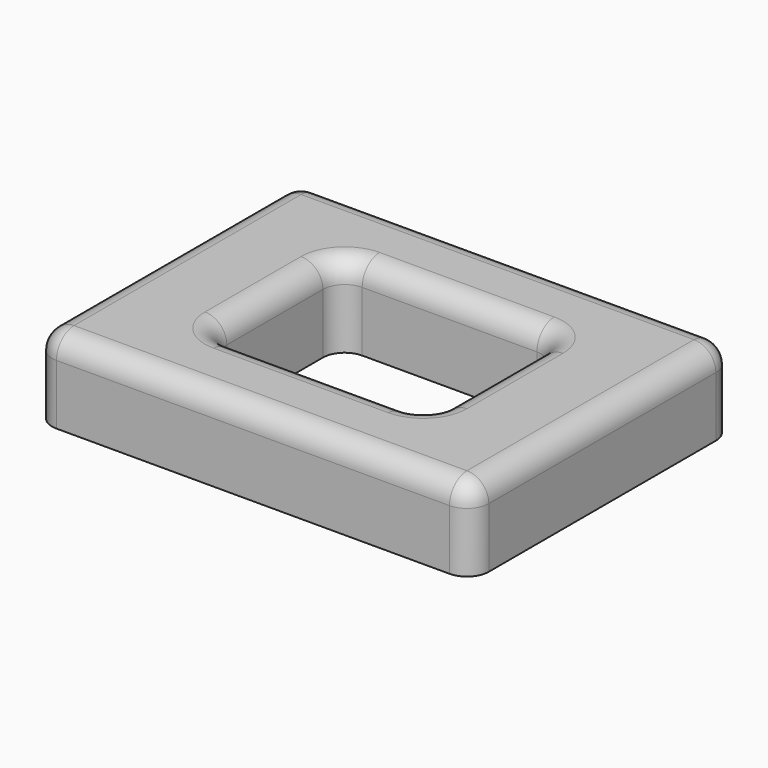
from build123d import *

# Parameters (mm, degrees)
F0_W     = 101.6
F0_H     = 76.2
F1_DEPTH = 19.05
F2_W     = 50.8
F2_H     = 38.1
F3_DEPTH = 25.4
F4_R     = 5.08


with BuildPart() as f1:
    # F0 (on Top) → F1 (new body)
    with BuildSketch(Plane.XY):
        Rectangle(F0_W, F0_H)
    extrude(amount=F1_DEPTH)

    # F2 (on face) → F3 (cut)
    with BuildSketch(Plane.XY.offset(19.05)):
        Rectangle(F2_W, F2_H)
    extrude(amount=-F3_DEPTH, mode=Mode.SUBTRACT)

    # F4
    f4_edges = [f1.edges().sort_by_distance(p)[0] for p in [
        (-50.8, 38.1, 9.525),
        (-50.8, -38.1, 9.525),
        (50.8, 38.1, 9.525),
        (25.4, -19.05, 9.525),
        (-25.4, 19.05, 9.525),
        (50.8, -38.1, 9.525),
        (-25.4, -19.05, 9.525),
        (-25.4, 0, 19.05),
        (-50.8, 0, 19.05),
        (0, -38.1, 19.05),
        (50.8, 0, 19.05),
        (0, 38.1, 19.05),
        (25.4, 19.05, 9.525),
        (0, -19.05, 19.05),
        (25.4, 0, 19.05),
        (0, 19.05, 19.05),
    ]]
    fillet(f4_edges, radius=F4_R)


solid = f1.part
